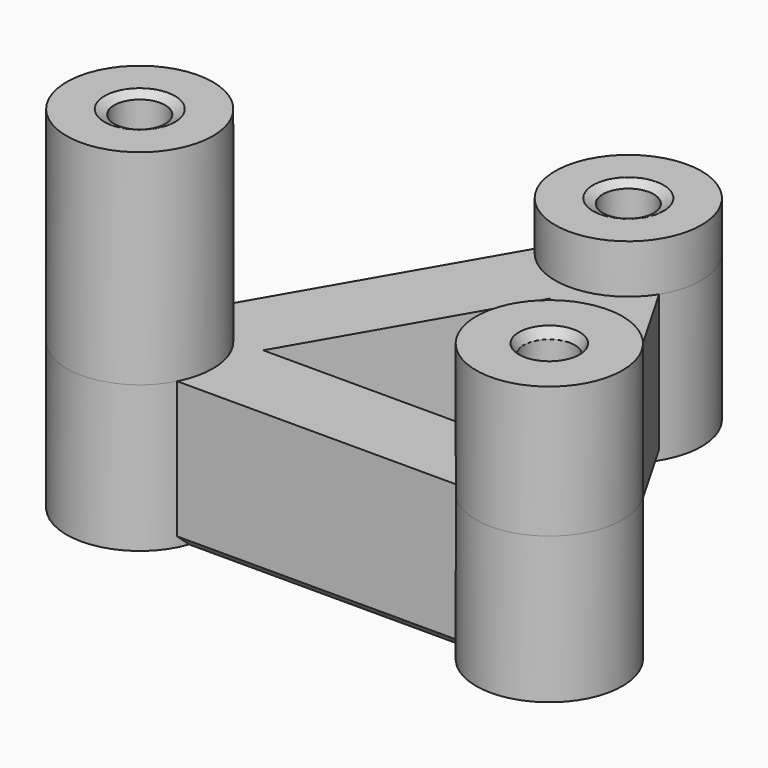
from build123d import *

# Parameters (mm, degrees)
F0_R        = 2.61
F1_DEPTH    = 15
F2_R        = 7.5
F2_R_2      = 2.61
F3_DEPTH    = 5
F4_R        = 7.5
F4_R_2      = 2.61
F5_DEPTH    = 13.5
F6_R        = 7.5
F6_R_2      = 2.61
F7_DEPTH    = 21
F8_C1_SIZE2 = 0.5
F8_C1_SIZE  = 1
F8_C2_SIZE2 = 0.5
F8_C2_SIZE  = 1
F8_C3_SIZE2 = 1
F8_C3_SIZE  = 0.5
F8_C4_SIZE2 = 1
F8_C4_SIZE  = 0.5
F8_C5_SIZE2 = 1
F8_C5_SIZE  = 0.5
F8_C6_SIZE2 = 0.5
F8_C6_SIZE  = 1
F9_SIZE     = 1


with BuildPart() as f1:
    # F0 (on Top) → F1 (new body)
    with BuildSketch(Plane.XY):
        with BuildLine():
            Line((20.7144641229, 7.4945626465), (6.3477137036, 32.3785043124))
            ThreePointArc((6.3477137036, 32.3785043124), (0, 43.8730669589), (-6.3477137036, 32.3785043124))
            Line((-6.3477137036, 32.3785043124), (-20.7144641229, 7.4945626465))
            ThreePointArc((-20.7144641229, 7.4945626465), (-27.4951905284, -3.75), (-14.3667504193, -3.5))
            Line((-14.3667504193, -3.5), (14.3667504193, -3.5))
            ThreePointArc((14.3667504193, -3.5), (27.4951905284, -3.75), (20.7144641229, 7.4945626465))
        make_face()
        with Locations((-21, 0)):
            Circle(F0_R, mode=Mode.SUBTRACT)
        with Locations((21, 0)):
            Circle(F0_R, mode=Mode.SUBTRACT)
        Polygon((12.3397459622, 5), (-12.3397459622, 5), (0, 26.3730669589), align=None, mode=Mode.SUBTRACT)
        with Locations((0, 36.3730669589)):
            Circle(F0_R, mode=Mode.SUBTRACT)
    extrude(amount=F1_DEPTH)

    # F2 (on face) → F3 (join)
    with BuildSketch(Plane.XY.offset(15)):
        with Locations((0, 36.3730669589)):
            Circle(F2_R)
        with Locations((0, 36.3730669589)):
            Circle(F2_R_2, mode=Mode.SUBTRACT)
    extrude(amount=F3_DEPTH)

    # F4 (on face) → F5 (join)
    with BuildSketch(Plane.XY.offset(15)):
        with Locations((21, 0)):
            Circle(F4_R)
        with Locations((21, 0)):
            Circle(F4_R_2, mode=Mode.SUBTRACT)
    extrude(amount=F5_DEPTH)

    # F6 (on face) → F7 (join)
    with BuildSketch(Plane.XY.offset(15)):
        with Locations((-21, 0)):
            Circle(F6_R)
        with Locations((-21, 0)):
            Circle(F6_R_2, mode=Mode.SUBTRACT)
    extrude(amount=F7_DEPTH)

    # F8: chamfer of 0.5 x 1 on 6 edges, made by hand

    # F8_c1
    f8_c1_edges = [f1.edges().sort_by_distance(p)[0] for p in [
        (-23.61, 0, 36),
    ]]
    f8_c1_side = f1.faces().sort_by_distance((-23.62, 0, 36))[0]
    chamfer(f8_c1_edges, length=F8_C1_SIZE, length2=F8_C1_SIZE2, reference=f8_c1_side)

    # F8_c2
    f8_c2_edges = [f1.edges().sort_by_distance(p)[0] for p in [
        (-23.61, 0, 0),
    ]]
    f8_c2_side = f1.faces().sort_by_distance((-23.61, 0, 0.01))[0]
    chamfer(f8_c2_edges, length=F8_C2_SIZE, length2=F8_C2_SIZE2, reference=f8_c2_side)

    # F8_c3
    f8_c3_edges = [f1.edges().sort_by_distance(p)[0] for p in [
        (18.39, 0, 0),
    ]]
    f8_c3_side = f1.faces().sort_by_distance((18.38, 0, 0))[0]
    chamfer(f8_c3_edges, length=F8_C3_SIZE, length2=F8_C3_SIZE2, reference=f8_c3_side)

    # F8_c4
    f8_c4_edges = [f1.edges().sort_by_distance(p)[0] for p in [
        (-2.61, 36.3730669589, 0),
    ]]
    f8_c4_side = f1.faces().sort_by_distance((-2.62, 36.3730669589, 0))[0]
    chamfer(f8_c4_edges, length=F8_C4_SIZE, length2=F8_C4_SIZE2, reference=f8_c4_side)

    # F8_c5
    f8_c5_edges = [f1.edges().sort_by_distance(p)[0] for p in [
        (-2.61, 36.3730669589, 20),
    ]]
    f8_c5_side = f1.faces().sort_by_distance((-2.61, 36.3730669589, 19.99))[0]
    chamfer(f8_c5_edges, length=F8_C5_SIZE, length2=F8_C5_SIZE2, reference=f8_c5_side)

    # F8_c6
    f8_c6_edges = [f1.edges().sort_by_distance(p)[0] for p in [
        (18.39, 0, 28.5),
    ]]
    f8_c6_side = f1.faces().sort_by_distance((18.39, 0, 28.49))[0]
    chamfer(f8_c6_edges, length=F8_C6_SIZE, length2=F8_C6_SIZE2, reference=f8_c6_side)

    # F9
    f9_edges = [f1.edges().sort_by_distance(p)[0] for p in [
        (6.169873, 15.686533, 0),
        (0, 5, 0),
        (-6.169873, 15.686533, 0),
        (0, -3.5, 0),
        (-13.531089, 19.936533, 0),
        (13.531089, 19.936533, 0),
    ]]
    chamfer(f9_edges, length=F9_SIZE)


solid = f1.part
